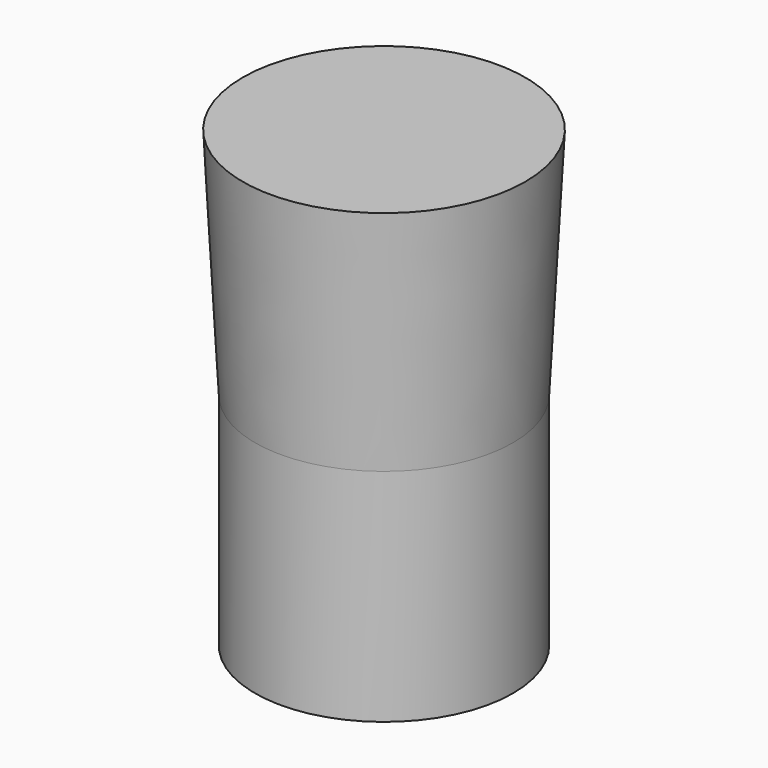
from build123d import *

# Parameters (mm, degrees)
F0_R          = 29.7196634515
F1_DEPTH      = 53.848
F1_TAPER      = -3
F1_DEPTH_BACK = 50.8


# Not quite as in the source:
# - the program builds the solid bodies; features that only make, move or delete a surface that nothing else refers to are left out


with BuildPart() as f1:
    # F0 (on Top) → F1 (new body, two sides)
    with BuildSketch(Plane.XY) as f1_sk:
        with Locations((-128.689289093, 17.6048204303)):
            Circle(F0_R)
    extrude(amount=F1_DEPTH, taper=F1_TAPER)
    extrude(f1_sk.sketch, amount=-F1_DEPTH_BACK)


solid = f1.part
